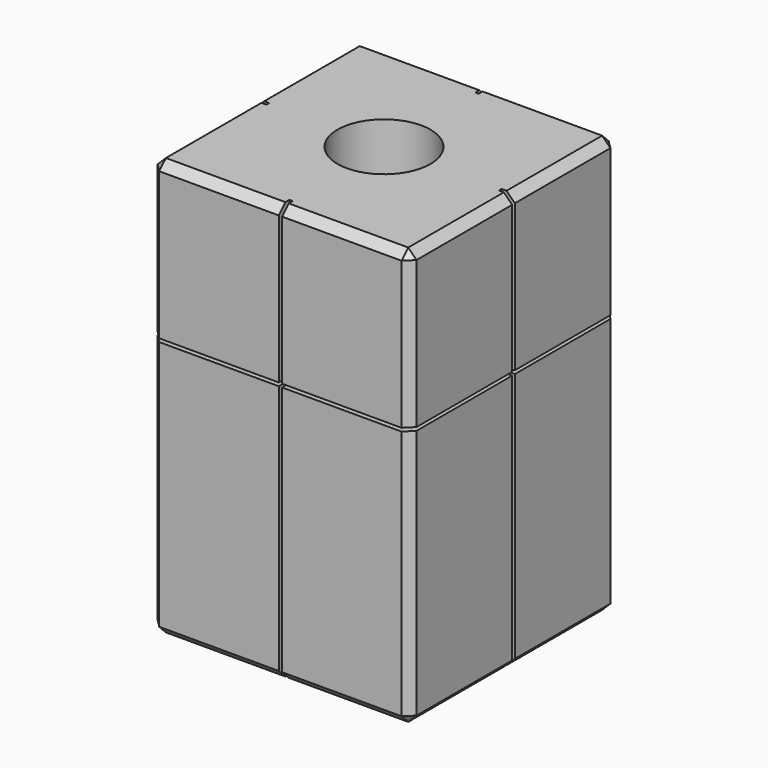
from build123d import *

# Parameters (mm, degrees)
F0_W            = 19.812
F0_H            = 19.812
F1_DEPTH        = 31.9532
F2_R            = 3.556
F3_DEPTH        = 25.9334
F4_T1_DEPTH     = 0.8065583261
F4_T3_DEPTH     = 0.8065583261
F4_T5_DEPTH     = 0.8065583261
F4_T7_DEPTH     = 0.8065583261
F4_T9_DEPTH     = 0.8065583261
F4_T11_DEPTH    = 0.8065583261
F4_T13_DEPTH    = 0.8065583261
F4_T15_DEPTH    = 0.8065583261
F4_T17_DEPTH    = 35.2192373947
F4_T19_DEPTH    = 23.0780373947
F4_T21_DEPTH    = 23.0780373947
F5_W            = 0.254
F5_H            = 11.8872
F5_H_2          = 0.254
F5_W_2          = 9.779
F5_H_3          = 19.812
F6_DEPTH        = 1.016
F6_COPIES_COUNT = 4
F7_W            = 0.254
F7_H            = 8.763
F7_H_2          = 0.254
F7_W_2          = 8.763
F8_DEPTH        = 1.016


# Not quite as in the source:
# - a fillet or chamfer that OpenCascade refuses, or shapes differently, is made with other operations: its cross-section is extruded or revolved along the edge and cut away or added
# - a pattern or mirror of a feature is missing from the dataset's text; its kind, count and spacing are read off the source's solid


with BuildPart() as f1:
    # F0 (on Top) → F1 (new body)
    with BuildSketch(Plane.XY):
        Rectangle(F0_W, F0_H)
    extrude(amount=F1_DEPTH)

    # F2 (on face) → F3 (cut)
    with BuildSketch(Plane.XY.offset(31.9532)):
        Circle(F2_R)
    extrude(amount=-F3_DEPTH, mode=Mode.SUBTRACT)

    # F4: chamfer of 0.635 on 12 edges, made by hand

    # F4_s2 → F4_t1 (cut)
    with BuildSketch(Plane(origin=(-6.1806666667, 6.1806666667, -6.1806666667), x_dir=(-0.7071067812, -0.7071067812, 0), z_dir=(-0.5773502692, 0.5773502692, -0.5773502692))):
        Polygon((-0.4490128061, 8.3474527951), (0, 7.5697398018), (0.4490128061, 8.3474527951), align=None)
    extrude(amount=F4_T1_DEPTH, mode=Mode.SUBTRACT)

    # F4_s4 → F4_t3 (cut)
    with BuildSketch(Plane(origin=(-16.8317333333, 16.8317333333, 16.8317333333), x_dir=(-0.7071067812, -0.7071067812, 0), z_dir=(-0.5773502692, 0.5773502692, 0.5773502692))):
        Polygon((-0.4490128061, 17.7422257546), (0, 18.5199387479), (0.4490128061, 17.7422257546), align=None)
    extrude(amount=F4_T3_DEPTH, mode=Mode.SUBTRACT)

    # F4_s6 → F4_t5 (cut)
    with BuildSketch(Plane(origin=(-6.1806666667, -6.1806666667, -6.1806666667), x_dir=(0.7071067812, -0.7071067812, 0), z_dir=(-0.5773502692, -0.5773502692, -0.5773502692))):
        Polygon((0.4490128061, 8.3474527951), (0, 7.5697398018), (-0.4490128061, 8.3474527951), align=None)
    extrude(amount=F4_T5_DEPTH, mode=Mode.SUBTRACT)

    # F4_s8 → F4_t7 (cut)
    with BuildSketch(Plane(origin=(-16.8317333333, -16.8317333333, 16.8317333333), x_dir=(0.7071067812, -0.7071067812, 0), z_dir=(-0.5773502692, -0.5773502692, 0.5773502692))):
        Polygon((0.4490128061, 17.7422257546), (0, 18.5199387479), (-0.4490128061, 17.7422257546), align=None)
    extrude(amount=F4_T7_DEPTH, mode=Mode.SUBTRACT)

    # F4_s10 → F4_t9 (cut)
    with BuildSketch(Plane(origin=(6.1806666667, -6.1806666667, -6.1806666667), x_dir=(0.7071067812, 0.7071067812, 0), z_dir=(0.5773502692, -0.5773502692, -0.5773502692))):
        Polygon((0.4490128061, 8.3474527951), (-0.4490128061, 8.3474527951), (0, 7.5697398018), align=None)
    extrude(amount=F4_T9_DEPTH, mode=Mode.SUBTRACT)

    # F4_s12 → F4_t11 (cut)
    with BuildSketch(Plane(origin=(16.8317333333, -16.8317333333, 16.8317333333), x_dir=(0.7071067812, 0.7071067812, 0), z_dir=(0.5773502692, -0.5773502692, 0.5773502692))):
        Polygon((0.4490128061, 17.7422257546), (-0.4490128061, 17.7422257546), (0, 18.5199387479), align=None)
    extrude(amount=F4_T11_DEPTH, mode=Mode.SUBTRACT)

    # F4_s14 → F4_t13 (cut)
    with BuildSketch(Plane(origin=(6.1806666667, 6.1806666667, -6.1806666667), x_dir=(-0.7071067812, 0.7071067812, 0), z_dir=(0.5773502692, 0.5773502692, -0.5773502692))):
        Polygon((-0.4490128061, 8.3474527951), (0.4490128061, 8.3474527951), (0, 7.5697398018), align=None)
    extrude(amount=F4_T13_DEPTH, mode=Mode.SUBTRACT)

    # F4_s16 → F4_t15 (cut)
    with BuildSketch(Plane(origin=(16.8317333333, 16.8317333333, 16.8317333333), x_dir=(-0.7071067812, 0.7071067812, 0), z_dir=(0.5773502692, 0.5773502692, 0.5773502692))):
        Polygon((-0.4490128061, 17.7422257546), (0.4490128061, 17.7422257546), (0, 18.5199387479), align=None)
    extrude(amount=F4_T15_DEPTH, mode=Mode.SUBTRACT)

    # F4_s18 → F4_t17 (cut)
    with BuildSketch(Plane.XY.offset(-1.6330186974)):
        Polygon((-9.271, 9.906), (-9.906, 9.271), (-9.906, 9.906), align=None)
        Polygon((-9.271, -9.906), (-9.906, -9.271), (-9.906, -9.906), align=None)
        Polygon((9.906, -9.271), (9.271, -9.906), (9.906, -9.906), align=None)
        Polygon((9.906, 9.271), (9.271, 9.906), (9.906, 9.906), align=None)
    extrude(amount=F4_T17_DEPTH, mode=Mode.SUBTRACT)

    # F4_s20 → F4_t19 (cut)
    with BuildSketch(Plane.XZ.offset(-11.5390186974)):
        Polygon((9.906, 31.3182), (9.271, 31.9532), (9.906, 31.9532), align=None)
        Polygon((-9.271, 31.9532), (-9.906, 31.3182), (-9.906, 31.9532), align=None)
        Polygon((9.906, 0.635), (9.271, 0), (9.906, 0), align=None)
        Polygon((-9.271, 0), (-9.906, 0.635), (-9.906, 0), align=None)
    extrude(amount=F4_T19_DEPTH, mode=Mode.SUBTRACT)

    # F4_s22 → F4_t21 (cut)
    with BuildSketch(Plane.YZ.offset(-11.5390186974)):
        Polygon((-9.906, 31.3182), (-9.271, 31.9532), (-9.906, 31.9532), align=None)
        Polygon((9.906, 31.3182), (9.271, 31.9532), (9.906, 31.9532), align=None)
        Polygon((9.906, 0.635), (9.271, 0), (9.906, 0), align=None)
        Polygon((-9.906, 0.635), (-9.271, 0), (-9.906, 0), align=None)
    extrude(amount=F4_T21_DEPTH, mode=Mode.SUBTRACT)

    # F5 (on face) → F6 (cut)
    with BuildSketch(Plane.XZ.offset(9.906)):
        with Locations((0, 26.0096)):
            Rectangle(F5_W, F5_H)
        with Locations((0, 19.939)):
            Rectangle(F5_W, F5_H_2)
        with Locations((-5.0165, 19.939)):
            Rectangle(F5_W_2, F5_H_2)
        with Locations((5.0165, 19.939)):
            Rectangle(F5_W_2, F5_H_2)
        with Locations((0, 9.906)):
            Rectangle(F5_W, F5_H_3)
    f6 = extrude(amount=-F6_DEPTH, mode=Mode.SUBTRACT)

    # F6_copies: F6 ×4 about axis
    f6_copies_axis = Axis((0, 0, 0), (0, 0, 1))
    for i in range(1, F6_COPIES_COUNT):
        add(f6.rotate(f6_copies_axis, i * 360 / F6_COPIES_COUNT), mode=Mode.SUBTRACT)

    # F7 (on face) → F8 (cut)
    with BuildSketch(Plane(origin=(0, 0, 0), x_dir=(1, 0, 0), z_dir=(0, 0, -1))):
        with Locations((0, 4.5085)):
            Rectangle(F7_W, F7_H)
        Rectangle(F7_W, F7_H_2)
        with Locations((-4.5085, 0)):
            Rectangle(F7_W_2, F7_H_2)
        with Locations((4.5085, 0)):
            Rectangle(F7_W_2, F7_H_2)
        with Locations((0, -4.5085)):
            Rectangle(F7_W, F7_H)
    extrude(amount=-F8_DEPTH, mode=Mode.SUBTRACT)


solid = f1.part
